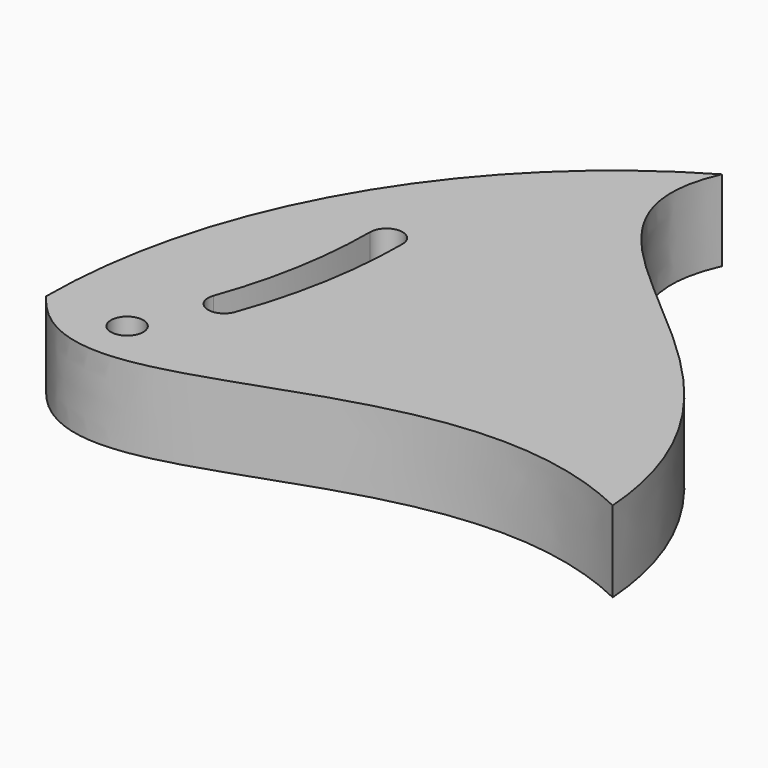
from build123d import *

# Parameters (mm, degrees)
F0_R     = 1
F1_DEPTH = 5


# Not quite as in the source:
# - ends of sketch curves that miss each other by under 0.0002 mm in the source are joined


with BuildPart() as f1:
    # F0 (on Top) → F1 (new body)
    with BuildSketch(Plane.XY):
        with BuildLine():
            add(Edge.make_bspline(
                [(12.5000001863, 30.3108888098), (7.72521306, 19.685755152), (28.7444061302, 17.0137217111), (30.0000001863, -3.226e-07)],
                knots=[0, 0, 0, 0, 35, 35, 35, 35], degree=3))
            ThreePointArc((12.5000001863, 30.3108888098), (-0.3108891325, 17.5), (-5, 0))
            add(Edge.make_bspline(
                [(-5, 0), (1.8142421031, -9.4476537779), (14.6378874779, 7.4194846675), (30.0000001863, -3.226e-07)],
                knots=[0, 0, 0, 0, 35, 35, 35, 35], degree=3))
        make_face()
        Circle(F0_R, mode=Mode.SUBTRACT)
        with BuildLine():
            ThreePointArc((3.1497091277, 4.3973755592), (1.867996364, 3.7997030808), (1.2703238856, 5.0814158445))
            ThreePointArc((1.2703238856, 5.0814158445), (2.5786627167, 9.9642028495), (3.0192378757, 15.0000000022))
            ThreePointArc((3.0192378757, 15.0000000022), (4.019237875, 16.0000000029), (5.0192378757, 15.0000000036))
            ThreePointArc((5.0192378757, 15.0000000036), (4.548278223, 9.6169064956), (3.1497091277, 4.3973755592))
        make_face(mode=Mode.SUBTRACT)
    extrude(amount=F1_DEPTH)


solid = f1.part
